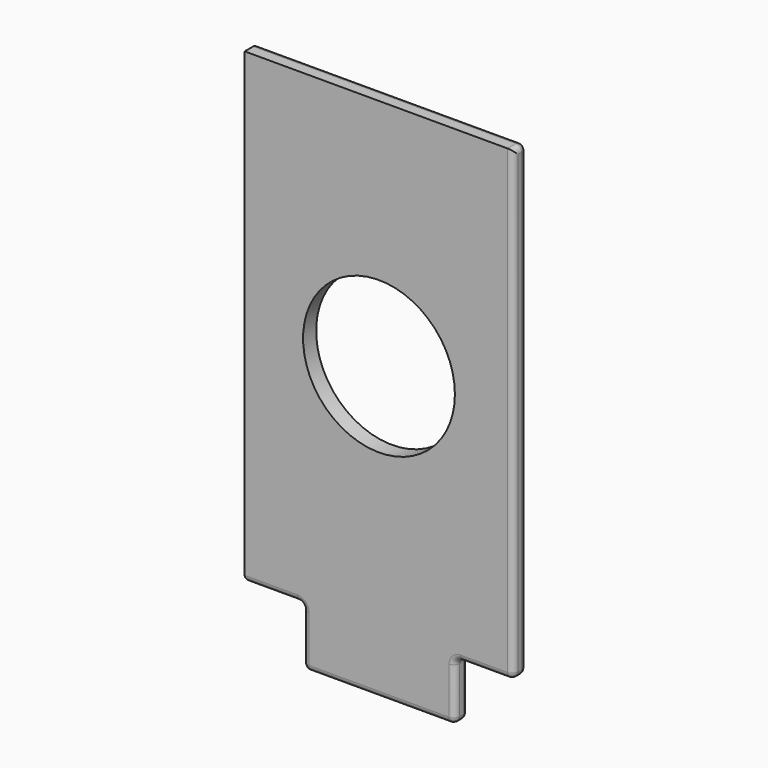
from build123d import *

# Parameters (mm, degrees)
F0_R     = 6.5
F1_DEPTH = 1.4
F2_W     = 15
F2_H     = 1
F3_DEPTH = 2
F4_R     = 0.49999


# Not quite as in the source:
# - a fillet or chamfer is up to 0.001 mm smaller than in the source, because OpenCascade refuses the exact size


with BuildPart() as f1:
    # F0 (on Front) → F1 (new body)
    with BuildSketch(Plane.XZ):
        Polygon((11.5, 20), (-11.5, 20), (-11.5, -20), (-6.5, -20), (-6.5, -25), (6.5, -25), (6.5, -20), (11.5, -20), align=None)
        Circle(F0_R, mode=Mode.SUBTRACT)
    extrude(amount=F1_DEPTH)

    # F2 (on face) → F3 (join)
    with BuildSketch(Plane(origin=(0, 0, 0), x_dir=(-1, 0, 0), z_dir=(0, 1, 0))):
        with Locations((0, 17.9)):
            Rectangle(F2_W, F2_H)
        with Locations((0, -17.9)):
            Rectangle(F2_W, F2_H)
    extrude(amount=F3_DEPTH)

    # F4 (radius 0.5 in the source; OpenCascade refuses exactly that, so slightly less here)
    f4_edges = [f1.edges().sort_by_distance(p)[0] for p in [
        (-6.5, -0.7, -25),
        (6.5, -0.7, -25),
        (0, 0, -25),
        (0, -1.4, -25),
        (6.5, -0.7, -20),
        (6.5, 0, -22.5),
        (6.5, -1.4, -22.5),
        (11.5, -0.7, -20),
        (11.5, -0.7, 20),
        (11.5, 0, 0),
        (11.5, -1.4, 0),
        (-11.5, 0, 0),
        (-6.5, -0.7, -20),
        (-6.5, 0, -22.5),
        (-6.5, -1.4, -22.5),
        (-11.5, -0.7, -20),
        (-9, 0, -20),
        (-9, -1.4, -20),
        (0, 0, 20),
        (0, 2, 17.4),
        (-7.5, 2, 17.9),
        (0, 2, 18.4),
        (7.5, 2, 17.9),
        (-7.5, 2, -17.9),
        (0, 2, -17.4),
        (7.5, 2, -17.9),
        (0, 2, -18.4),
        (9, 0, -20),
        (9, -1.4, -20),
    ]]
    fillet(f4_edges, radius=F4_R)


solid = f1.part
